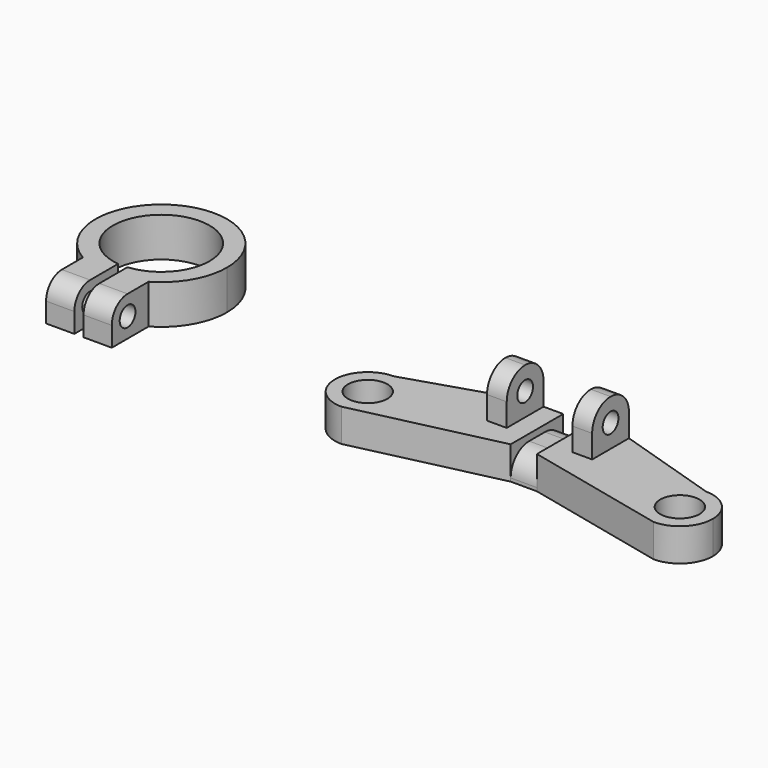
from build123d import *

# Parameters (mm, degrees)
F1_DEPTH = 6
F3_D     = 3
F4_W     = 3
F4_H     = 7
F5_DEPTH = 12
F4_R     = 3
F6_DEPTH = 5
F7_DEPTH = 4
F8_R     = 4.99999
F9_R     = 3.49999
F12_D    = 3
F13_R    = 3


# Not quite as in the source:
# - a fillet or chamfer is up to 0.001 mm smaller than in the source, because OpenCascade refuses the exact size
# - a feature names something its author has since deleted; it is built from what else it names


with BuildPart() as f1:
    # F0 (on Top) → F1 (new body)
    with BuildSketch(Plane.XY):
        with BuildLine():
            ThreePointArc((-26.4478022211, 9.2937625569), (-28.5229179157, 8.3913259797), (-30.7478022211, 7.978546681))
            Line((-30.7478022211, 7.978546681), (-30.7478022211, 2.2937625569))
            Line((-30.7478022211, 2.2937625569), (-26.4478022211, 2.2937625569))
            Line((-26.4478022211, 2.2937625569), (-26.4478022211, 9.2937625569))
        make_face()
        with BuildLine():
            Line((-32.1478022211, 2.2937625569), (-32.1478022211, 7.978546681))
            ThreePointArc((-32.1478022211, 7.978546681), (-34.3726865265, 8.3913259797), (-36.4478022211, 9.2937625569))
            Line((-36.4478022211, 9.2937625569), (-36.4478022211, 2.2937625569))
            Line((-36.4478022211, 2.2937625569), (-32.1478022211, 2.2937625569))
        make_face()
        with BuildLine():
            ThreePointArc((-32.1478022211, 10.6374258586), (-36.3913586332, 23.3931111885), (-24.0978022211, 17.9540165948))
            ThreePointArc((-24.0978022211, 17.9540165948), (-26.0087076273, 13.0104601826), (-30.7478022211, 10.6374258586))
            Line((-30.7478022211, 10.6374258586), (-30.7478022211, 7.978546681))
            ThreePointArc((-30.7478022211, 7.978546681), (-28.5229179157, 8.3913259797), (-26.4478022211, 9.2937625569))
            ThreePointArc((-26.4478022211, 9.2937625569), (-22.7875481833, 12.9540165948), (-21.4478022211, 17.9540165948))
            ThreePointArc((-21.4478022211, 17.9540165948), (-36.4478022211, 26.6142706326), (-36.4478022211, 9.2937625569))
            ThreePointArc((-36.4478022211, 9.2937625569), (-34.3726865265, 8.3913259797), (-32.1478022211, 7.978546681))
            Line((-32.1478022211, 7.978546681), (-32.1478022211, 10.6374258586))
        make_face()
    extrude(amount=F1_DEPTH)

    # F3 (through all)
    with Locations(Plane.YZ.offset(-26.4478022211)):
        with Locations((5.2937625569, 3)):
            Hole(F3_D / 2)

    # F13
    f13_edges = [f1.edges().sort_by_distance(p)[0] for p in [
        (-34.297802, 2.293763, 6),
        (-28.597802, 2.293763, 6),
    ]]
    fillet(f13_edges, radius=F13_R)


with BuildPart() as f5:
    # F4 (on Top) → F5 (new body)
    with BuildSketch(Plane.XY):
        with Locations((27.5828619152, 11.5)):
            Rectangle(F4_W, F4_H)
    extrude(amount=F5_DEPTH)

    # F4 (on Top) → F6 (join)
    with BuildSketch(Plane.XY):
        Polygon((10.3328619152, 10), (5.3328619152, 10), (5.3328619152, 0), (10.3328619152, 0), (32.0828619152, 5), (32.0828619152, 8), (29.0828619152, 8), (26.0828619152, 8), (26.0828619152, 15), align=None)
        with Locations((10.3328619152, 5)):
            Circle(F4_R, mode=Mode.SUBTRACT)
        with Locations((30.5828619152, 11.5)):
            Rectangle(F4_W, F4_H)
    extrude(amount=F6_DEPTH)

    # F4 (on Top) → F7 (join)
    with BuildSketch(Plane.XY):
        Polygon((32.0828619152, 8), (32.0828619152, 5), (34.0828619152, 5), (34.0828619152, 15), (32.0828619152, 15), align=None)
    extrude(amount=F7_DEPTH)

    # F8 (radius 5 in the source; OpenCascade refuses exactly that, so slightly less here)
    f8_edges = [f5.edges().sort_by_distance(p)[0] for p in [
        (5.332862, 0, 2.5),
        (5.332862, 10, 2.5),
    ]]
    fillet(f8_edges, radius=F8_R)

    # F9 (radius 3.5 in the source; OpenCascade refuses exactly that, so slightly less here)
    f9_edges = [f5.edges().sort_by_distance(p)[0] for p in [
        (33.082862, 15, 4),
        (33.082862, 5, 4),
        (27.582862, 15, 12),
        (27.582862, 8, 12),
    ]]
    fillet(f9_edges, radius=F9_R)

    # F11: F5 across face


with BuildPart() as f5_1:
    add(f5.part)
    add(f5.part.mirror(Plane(origin=(34.0828619152, 10, 1.8156418236), x_dir=(0, 1, 0), z_dir=(1, 0, 0))))

    # F12 (through all)
    with Locations(Plane(origin=(26.0828619152, 0, 0), x_dir=(0, -1, 0), z_dir=(-1, 0, 0))):
        with Locations((-11.5, 8.5)):
            Hole(F12_D / 2)


solid = Compound([f1.part, f5_1.part])
